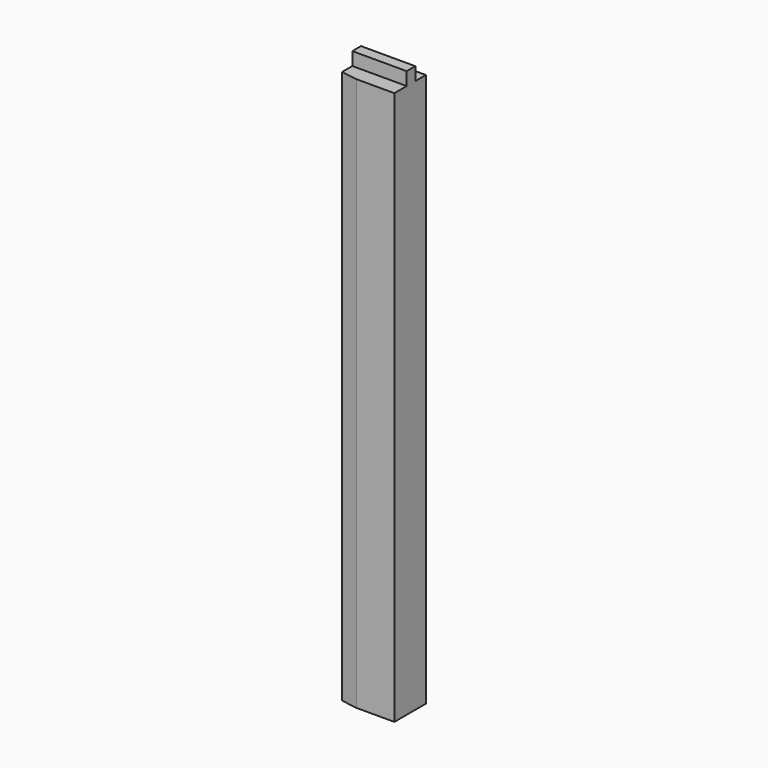
from build123d import *

# Parameters (mm, degrees)
F0_W     = 105.0320863724
F0_H     = 79.1744627059
F1_DEPTH = 76.2
F2_DEPTH = 990.6
F3_W     = 105.0320863724
F3_H     = 20.9305938333
F4_DEPTH = 25.4
F5_SIZE2 = 5.0287059803
F5_SIZE  = 31.75
F6_SIZE2 = 5.0287059803
F6_SIZE  = 31.75


# Not quite as in the source:
# - the program builds the solid bodies; features that only make, move or delete a surface that nothing else refers to are left out


with BuildPart() as f1:
    # F0 (on Front) → F1 (new body)
    with BuildSketch(Plane.XZ):
        with Locations((5.5860057473, -1.434026286)):
            Rectangle(F0_W, F0_H)
    extrude(amount=F1_DEPTH)

    # F2 (add): a face of the model
    f2_faces = [f1.faces().sort_by_distance(p)[0] for p in [
        (5.5860057473, -38.1, 38.1532050669),
    ]]
    extrude(f2_faces, amount=F2_DEPTH)

    # F3 (on face) → F4 (join)
    with BuildSketch(Plane.XY.offset(1028.7532050669)):
        with Locations((5.5860057473, -36.0199743882)):
            Rectangle(F3_W, F3_H)
    extrude(amount=F4_DEPTH)

    # F5
    f5_edges = [f1.edges().sort_by_distance(p)[0] for p in [
        (-46.930037, -76.2, 493.865974),
    ]]
    f5_side = f1.faces().sort_by_distance((5.586006, -76.2, 493.865974))[0]
    chamfer(f5_edges, length=F5_SIZE, length2=F5_SIZE2, reference=f5_side)

    # F6
    f6_edges = [f1.edges().sort_by_distance(p)[0] for p in [
        (-46.930037, 0, 493.865974),
    ]]
    f6_side = f1.faces().sort_by_distance((5.586006, 0, 493.865974))[0]
    chamfer(f6_edges, length=F6_SIZE, length2=F6_SIZE2, reference=f6_side)


solid = f1.part
